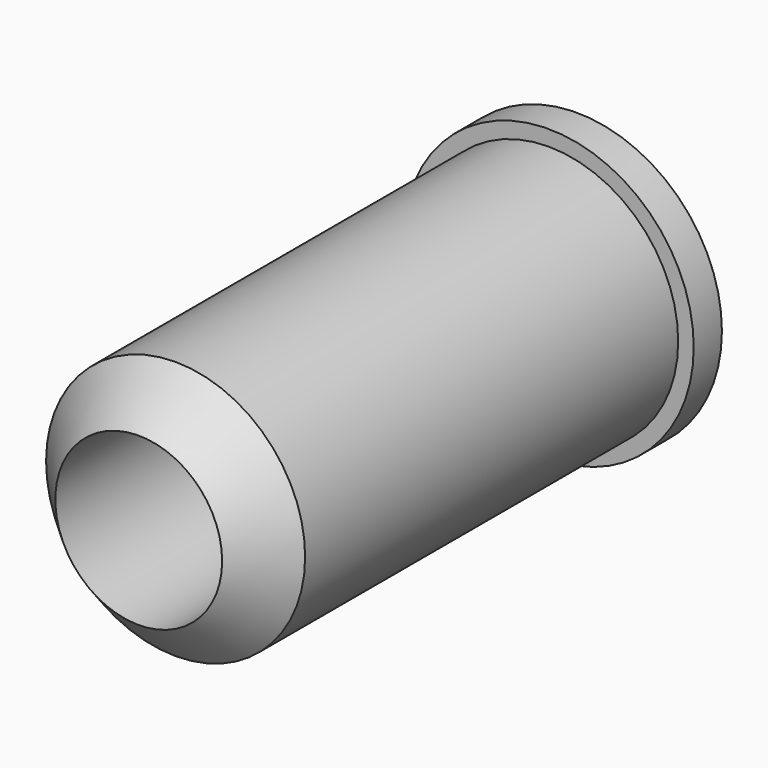
from build123d import *

# Parameters (mm, degrees)
F0_R      = 14
F1_DEPTH  = 3.4
F3_R      = 12.5
F4_DEPTH  = 50
F6_R      = 8.05
F7_DEPTH  = 40
F9_R      = 6.25
F10_DEPTH = 66.1


# Not quite as in the source:
# - a fillet or chamfer that OpenCascade refuses, or shapes differently, is made with other operations: its cross-section is extruded or revolved along the edge and cut away or added


with BuildPart() as f1:
    # F0 (on Front) → F1 (new body)
    with BuildSketch(Plane.XZ):
        Circle(F0_R)
    extrude(amount=F1_DEPTH)

    # F3 (on offset) → F4 (join)
    with BuildSketch(Plane.XZ.offset(3.4)):
        Circle(F3_R)
    extrude(amount=F4_DEPTH)

    # F6 (on offset) → F7 (cut)
    with BuildSketch(Plane.XZ.offset(53.4)):
        Circle(F6_R)
    extrude(amount=-F7_DEPTH, mode=Mode.SUBTRACT)

    # F8: chamfer of 5 on 1 edges, made by hand

    # F8_s1 → F8_t2 (revolve, cut)
    with BuildSketch(Plane.XY):
        Polygon((12.5, -48.4), (7.5, -53.4), (12.5, -53.4), align=None)
    revolve(axis=Axis((0, -53.4, 0), (0, -1, 0)), mode=Mode.SUBTRACT)

    # F9 (on Front) → F10 (cut)
    with BuildSketch(Plane.XZ):
        Circle(F9_R)
    extrude(amount=F10_DEPTH, mode=Mode.SUBTRACT)


solid = f1.part
